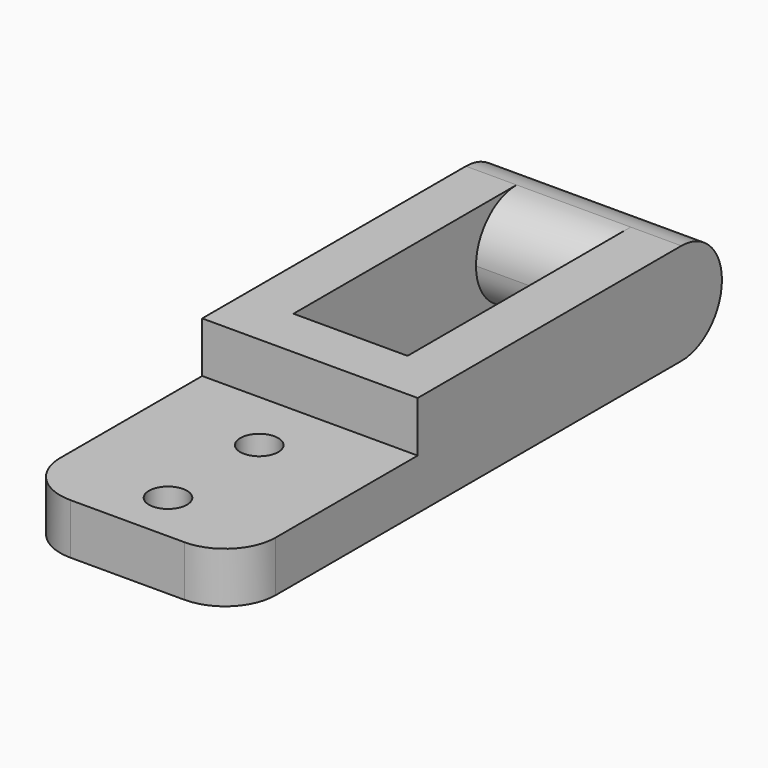
from build123d import *

# Parameters (mm, degrees)
F2_W         = 17
F2_H         = 48
F2_R         = 1.5
F2_W_2       = 9
F2_H_2       = 18
F3_DEPTH     = 4
F4_W         = 17
F4_H         = 30
F4_W_2       = 9
F4_H_2       = 18
F5_DEPTH     = 4
F6_R         = 3.99999
F7_TEXT_SIZE = 2.7777777778
F8_DEPTH     = 0.5


# Not quite as in the source:
# - a fillet or chamfer is up to 0.001 mm smaller than in the source, because OpenCascade refuses the exact size
# - Text() gives the source's letters only with a copy of the font that has no kerning and outlines rounded to 1/6400 em; it was checked with that copy


with BuildPart() as f3:
    # F2 (on Top) → F3 (new body)
    with BuildSketch(Plane.XY):
        Rectangle(F2_W, F2_H)
        with Locations((0, -20)):
            Circle(F2_R, mode=Mode.SUBTRACT)
        with Locations((0, -11)):
            Circle(F2_R, mode=Mode.SUBTRACT)
        with Locations((0, 7)):
            Rectangle(F2_W_2, F2_H_2, mode=Mode.SUBTRACT)
    extrude(amount=F3_DEPTH)

    # F4 (on face) → F5 (join)
    with BuildSketch(Plane.XY.offset(4)):
        with Locations((0, 9)):
            Rectangle(F4_W, F4_H)
        with Locations((0, 7)):
            Rectangle(F4_W_2, F4_H_2, mode=Mode.SUBTRACT)
    extrude(amount=F5_DEPTH)

    # F6 (radius 4 in the source; OpenCascade refuses exactly that, so slightly less here)
    f6_edges = [f3.edges().sort_by_distance(p)[0] for p in [
        (0, 16, 8),
        (0, 16, 0),
        (0, 24, 0),
        (0, 24, 8),
        (-8.5, -24, 2),
        (8.5, -24, 2),
        (0, -2, 0),
    ]]
    fillet(f6_edges, radius=F6_R)

    # F7 (on face) → F8 (cut)
    with BuildSketch(Plane(origin=(0, -2, 0), x_dir=(-1, 0, 0), z_dir=(0, 1, 0))):
        with Locations((-2.3786892361, 5)):
            Text('3E8', F7_TEXT_SIZE, font='Open Sans', text_align=(TextAlign.LEFT, TextAlign.BOTTOM))
    extrude(amount=-F8_DEPTH, mode=Mode.SUBTRACT)


solid = f3.part
